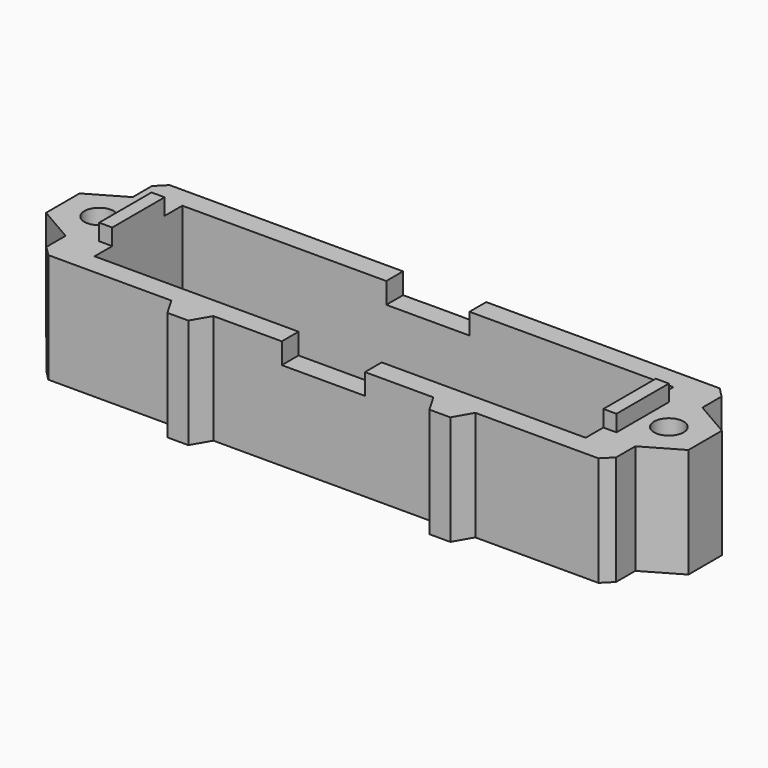
from build123d import *

# Parameters (mm, degrees)
F0_R     = 2.25
F0_W     = 75
F0_H     = 16.75
F1_DEPTH = 16.75
F2_SIZE  = 1.5
F3_W     = 3
F3_H     = 11
F4_DEPTH = 3
F5_W     = 2
F5_H     = 10
F6_DEPTH = 2.5
F7_W     = 12.7
F7_H     = 6.4
F8_DEPTH = 25.9222812921
F9_SIZE  = 2.75


with BuildPart() as f1:
    # F0 (on Top) → F1 (new body)
    with BuildSketch(Plane.XY):
        Polygon((43.5, 6.4), (43.5, 11.575), (3.2, 11.575), (1.6, 14.3462812921), (-1.6, 14.3462812921), (-3.2, 11.575), (-43.5, 11.575), (-43.5, 6.4), (-49.0425625842, 3.2), (-49.0425625842, -3.2), (-43.5, -6.4), (-43.5, -11.575), (-23.2, -11.575), (-21.6, -14.3462812921), (-18.4, -14.3462812921), (-16.8, -11.575), (16.8, -11.575), (18.4, -14.3462812921), (21.6, -14.3462812921), (23.2, -11.575), (43.5, -11.575), (43.5, -6.4), (49.0425625842, -3.2), (49.0425625842, 3.2), align=None)
        with Locations((-43.5, 0)):
            Circle(F0_R, mode=Mode.SUBTRACT)
        Rectangle(F0_W, F0_H, mode=Mode.SUBTRACT)
        with Locations((43.5, 0)):
            Circle(F0_R, mode=Mode.SUBTRACT)
    extrude(amount=F1_DEPTH)

    # F2
    f2_edges = [f1.edges().sort_by_distance(p)[0] for p in [
        (-43.5, 11.575, 8.375),
        (43.5, 11.575, 8.375),
        (43.5, -11.575, 8.375),
        (-43.5, -11.575, 8.375),
    ]]
    chamfer(f2_edges, length=F2_SIZE)

    # F3 (on Top) → F4 (cut)
    with BuildSketch(Plane.XY):
        with Locations((-39, 0)):
            Rectangle(F3_W, F3_H)
        with Locations((39, 0)):
            Rectangle(F3_W, F3_H)
    extrude(amount=F4_DEPTH, mode=Mode.SUBTRACT)

    # F5 (on face) → F6 (join)
    with BuildSketch(Plane.XY.offset(16.75)):
        with Locations((-38.5, 0)):
            Rectangle(F5_W, F5_H)
        with Locations((38.5, 0)):
            Rectangle(F5_W, F5_H)
    extrude(amount=F6_DEPTH)

    # F7 (on face) → F8 (cut, through all)
    with BuildSketch(Plane.XZ.offset(11.575)):
        with Locations((0, 16.75)):
            Rectangle(F7_W, F7_H)
    extrude(amount=-F8_DEPTH, mode=Mode.SUBTRACT)

    # F9
    f9_edges = [f1.edges().sort_by_distance(p)[0] for p in [
        (0, 14.346281, 13.55),
    ]]
    chamfer(f9_edges, length=F9_SIZE)


solid = f1.part
